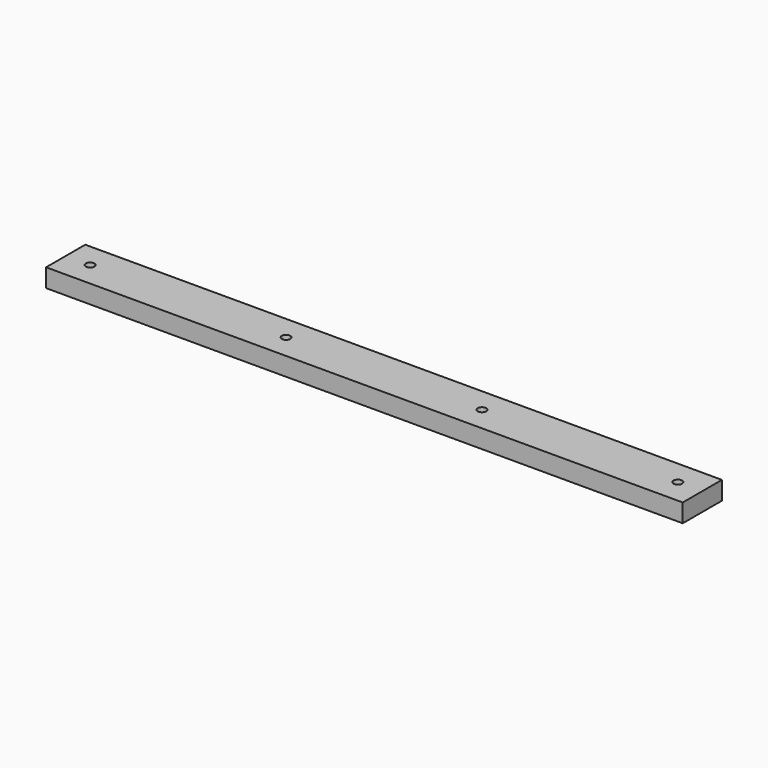
from build123d import *

# Parameters (mm, degrees)
F0_W           = 660.4
F0_H           = 50.8
F1_DEPTH       = 19.05
F2_D           = 8.89
F2_CBORE_D     = 12.065
F2_CBORE_DEPTH = 12.7


# Not quite as in the source:
# - a length typed as a fraction of an inch, garbled in the dataset ("3 / 203.2 mm" for 3/8 in), is restored


with BuildPart() as f1:
    # F0 (on Top) → F1 (new body)
    with BuildSketch(Plane.XY):
        with Locations((304.8, 0)):
            Rectangle(F0_W, F0_H)
    extrude(amount=F1_DEPTH)

    # F2 (through all)
    with Locations(Plane(origin=(0, 0, 0), x_dir=(1, 0, 0), z_dir=(0, 0, -1))):
        with Locations((0, 0), (203.2, 0), (406.4, 0), (609.6, 0)):
            CounterBoreHole(F2_D / 2, F2_CBORE_D / 2, F2_CBORE_DEPTH)


solid = f1.part
